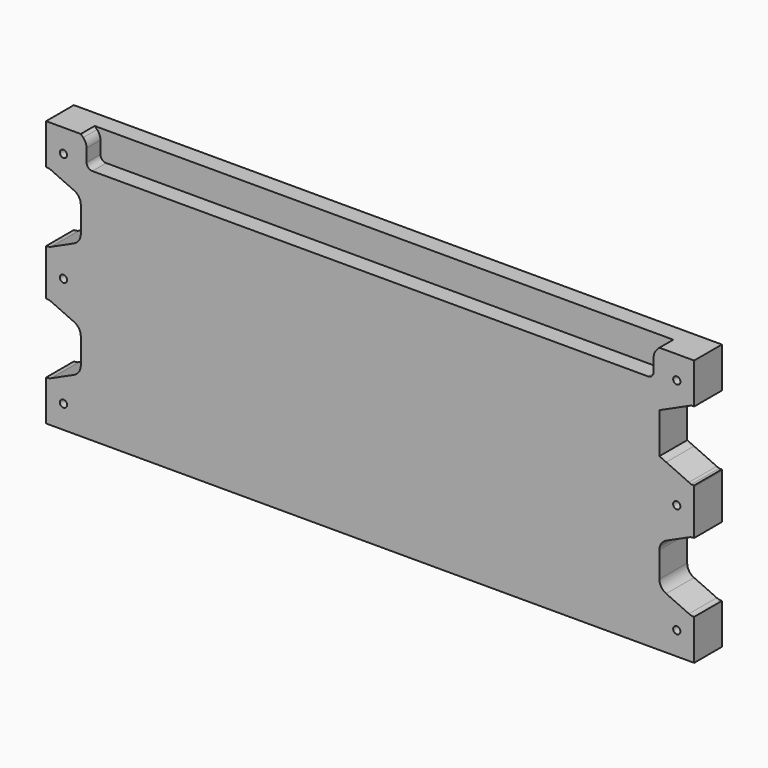
from build123d import *

# Parameters (mm, degrees)
F0_R     = 1.984375
F1_DEPTH = 9.525
F2_DEPTH = 9.525
F3_SIZE  = 3.175
F4_R     = 6.35


# Not quite as in the source:
# - ends of sketch curves that miss each other by under 0.0002 mm in the source are joined


with BuildPart() as f1:
    # F0 (on Front) → F1 (new body)
    with BuildSketch(Plane.XZ):
        with BuildLine():
            ThreePointArc((106.6892375248, 39.5968594302), (108.9343015551, 40.5267953999), (109.8642375248, 42.7718594302))
            Line((109.8642375248, 42.7718594302), (109.8642375248, 55.4718594302))
            Line((109.8642375248, 55.4718594302), (-201.2857624752, 55.4718594302))
            Line((-201.2857624752, 55.4718594302), (-201.2857624752, 42.7718594302))
            ThreePointArc((-201.2857624752, 42.7718594302), (-200.3558265055, 40.5267953999), (-198.1107624752, 39.5968594302))
            Line((-198.1107624752, 39.5968594302), (106.6892375248, 39.5968594302))
        make_face()
        with BuildLine():
            Line((109.8642375248, 55.4718594302), (109.8642375248, 42.7718594302))
            ThreePointArc((109.8642375248, 42.7718594302), (108.9343015551, 40.5267953999), (106.6892375248, 39.5968594302))
            Line((106.6892375248, 39.5968594302), (-198.1107624752, 39.5968594302))
            ThreePointArc((-198.1107624752, 39.5968594302), (-200.3558265055, 40.5267953999), (-201.2857624752, 42.7718594302))
            Line((-201.2857624752, 42.7718594302), (-201.2857624752, 55.4718594302))
            Line((-201.2857624752, 55.4718594302), (-223.5107624752, 55.4718594302))
            Line((-223.5107624752, 55.4718594302), (-223.5107624752, 33.2468594302))
            Line((-223.5107624752, 33.2468594302), (-223.2986885503, 33.2468594302))
            ThreePointArc((-223.2986885503, 33.2468594302), (-221.9543922864, 33.1029344825), (-220.6710339026, 32.6776838569))
            Line((-220.6710339026, 32.6776838569), (-208.1831078275, 27.0013383101))
            ThreePointArc((-208.1831078275, 27.0013383101), (-205.471843717, 24.6583106333), (-204.4607624752, 21.2205138834))
            Line((-204.4607624752, 21.2205138834), (-204.4607624752, 7.1731958926))
            ThreePointArc((-204.4607624752, 7.1731958926), (-205.4718446589, 3.7353976799), (-208.1831109951, 1.392370026))
            Line((-208.1831109951, 1.392370026), (-220.6710352489, -4.2839664363))
            ThreePointArc((-220.6710352489, -4.2839664363), (-221.9543921654, -4.7092159904), (-223.298686729, -4.8531405698))
            Line((-223.298686729, -4.8531405698), (-223.5107370752, -4.8531405698))
            Line((-223.5107370752, -4.8531405698), (-223.5107624752, -30.2531405698))
            Line((-223.5107624752, -30.2531405698), (-223.298686729, -30.2531405698))
            ThreePointArc((-223.298686729, -30.2531405698), (-221.9543921654, -30.3970651492), (-220.6710352489, -30.8223147033))
            Line((-220.6710352489, -30.8223147033), (-208.1831109951, -36.4986511657))
            ThreePointArc((-208.1831109951, -36.4986511657), (-205.4718446589, -38.8416788196), (-204.4607624752, -42.2794770322))
            Line((-204.4607624752, -42.2794770322), (-204.4607624752, -56.326795023))
            ThreePointArc((-204.4607624752, -56.326795023), (-205.471843717, -59.7645917729), (-208.1831078275, -62.1076194497))
            Line((-208.1831078275, -62.1076194497), (-220.6710339026, -67.7839649965))
            ThreePointArc((-220.6710339026, -67.7839649965), (-221.9543922864, -68.2092156221), (-223.2986885503, -68.3531405698))
            Line((-223.2986885503, -68.3531405698), (-223.5107370752, -68.3531405698))
            Line((-223.5107370752, -68.3531405698), (-223.5107624752, -90.5781405698))
            Line((-223.5107624752, -90.5781405698), (132.0892375248, -90.5781405698))
            Line((132.0892375248, -90.5781405698), (132.0892375248, -68.3531405698))
            Line((132.0892375248, -68.3531405698), (131.8771635999, -68.3531405698))
            ThreePointArc((131.8771635999, -68.3531405698), (130.532867336, -68.2092156221), (129.2495089522, -67.7839649965))
            Line((129.2495089522, -67.7839649965), (116.7615828771, -62.1076194497))
            ThreePointArc((116.7615828771, -62.1076194497), (114.0503187666, -59.7645917729), (113.0392375248, -56.326795023))
            Line((113.0392375248, -56.326795023), (113.0392375248, -42.2794770322))
            ThreePointArc((113.0392375248, -42.2794770322), (114.0503197085, -38.8416788196), (116.7615860447, -36.4986511657))
            Line((116.7615860447, -36.4986511657), (129.2495102985, -30.8223147033))
            ThreePointArc((129.2495102985, -30.8223147033), (130.5328672149, -30.3970651492), (131.8771617786, -30.2531405698))
            Line((131.8771617786, -30.2531405698), (132.0892121248, -30.2531405698))
            Line((132.0892121248, -30.2531405698), (132.0892375248, -5.5747531892))
            Line((132.0892375248, -5.5747531892), (130.5016917914, -4.8531405698))
            Line((130.5016917914, -4.8531405698), (129.2495102985, -4.2839664363))
            Line((129.2495102985, -4.2839664363), (116.7615860447, 1.392370026))
            Line((116.7615860447, 1.392370026), (113.0392375248, 3.0843487889))
            Line((113.0392375248, 3.0843487889), (113.0392375248, 7.1731958926))
            Line((113.0392375248, 7.1731958926), (113.0392375248, 21.2205138834))
            Line((113.0392375248, 21.2205138834), (113.0392375248, 25.3093700715))
            Line((113.0392375248, 25.3093700715), (116.7615794549, 27.001345839))
            Line((116.7615794549, 27.001345839), (129.2495086403, 32.677684543))
            Line((129.2495086403, 32.677684543), (130.5016917914, 33.2468594302))
            Line((130.5016917914, 33.2468594302), (132.0892375248, 33.9684720496))
            Line((132.0892375248, 33.9684720496), (132.0892375248, 55.4718594302))
            Line((132.0892375248, 55.4718594302), (109.8642375248, 55.4718594302))
        make_face()
        with Locations((-213.9857624752, -77.8781405698)):
            Circle(F0_R, mode=Mode.SUBTRACT)
        with Locations((122.5642375248, -77.8781405698)):
            Circle(F0_R, mode=Mode.SUBTRACT)
        with Locations((-213.9857624752, -17.5531402737)):
            Circle(F0_R, mode=Mode.SUBTRACT)
        with Locations((-213.9857624752, 42.7718594302)):
            Circle(F0_R, mode=Mode.SUBTRACT)
        with Locations((122.5642375248, -17.5531402737)):
            Circle(F0_R, mode=Mode.SUBTRACT)
        with Locations((122.5642375248, 42.7718594302)):
            Circle(F0_R, mode=Mode.SUBTRACT)
        Polygon((132.0892375248, 33.2468594302), (132.0892375248, 33.9684720496), (130.5016917914, 33.2468594302), (131.8771635999, 33.2468594302), align=None)
        Polygon((132.0892375248, -5.5747531892), (132.0892375248, -4.8531405698), (131.8771617786, -4.8531405698), (130.5016917914, -4.8531405698), align=None)
    extrude(amount=-F1_DEPTH)

    # F0 (on Front) → F2 (join)
    with BuildSketch(Plane.XZ):
        with BuildLine():
            Line((109.8642375248, 55.4718594302), (109.8642375248, 42.7718594302))
            ThreePointArc((109.8642375248, 42.7718594302), (108.9343015551, 40.5267953999), (106.6892375248, 39.5968594302))
            Line((106.6892375248, 39.5968594302), (-198.1107624752, 39.5968594302))
            ThreePointArc((-198.1107624752, 39.5968594302), (-200.3558265055, 40.5267953999), (-201.2857624752, 42.7718594302))
            Line((-201.2857624752, 42.7718594302), (-201.2857624752, 55.4718594302))
            Line((-201.2857624752, 55.4718594302), (-223.5107624752, 55.4718594302))
            Line((-223.5107624752, 55.4718594302), (-223.5107624752, 33.2468594302))
            Line((-223.5107624752, 33.2468594302), (-223.2986885503, 33.2468594302))
            ThreePointArc((-223.2986885503, 33.2468594302), (-221.9543922864, 33.1029344825), (-220.6710339026, 32.6776838569))
            Line((-220.6710339026, 32.6776838569), (-208.1831078275, 27.0013383101))
            ThreePointArc((-208.1831078275, 27.0013383101), (-205.471843717, 24.6583106333), (-204.4607624752, 21.2205138834))
            Line((-204.4607624752, 21.2205138834), (-204.4607624752, 7.1731958926))
            ThreePointArc((-204.4607624752, 7.1731958926), (-205.4718446589, 3.7353976799), (-208.1831109951, 1.392370026))
            Line((-208.1831109951, 1.392370026), (-220.6710352489, -4.2839664363))
            ThreePointArc((-220.6710352489, -4.2839664363), (-221.9543921654, -4.7092159904), (-223.298686729, -4.8531405698))
            Line((-223.298686729, -4.8531405698), (-223.5107370752, -4.8531405698))
            Line((-223.5107370752, -4.8531405698), (-223.5107624752, -30.2531405698))
            Line((-223.5107624752, -30.2531405698), (-223.298686729, -30.2531405698))
            ThreePointArc((-223.298686729, -30.2531405698), (-221.9543921654, -30.3970651492), (-220.6710352489, -30.8223147033))
            Line((-220.6710352489, -30.8223147033), (-208.1831109951, -36.4986511657))
            ThreePointArc((-208.1831109951, -36.4986511657), (-205.4718446589, -38.8416788196), (-204.4607624752, -42.2794770322))
            Line((-204.4607624752, -42.2794770322), (-204.4607624752, -56.326795023))
            ThreePointArc((-204.4607624752, -56.326795023), (-205.471843717, -59.7645917729), (-208.1831078275, -62.1076194497))
            Line((-208.1831078275, -62.1076194497), (-220.6710339026, -67.7839649965))
            ThreePointArc((-220.6710339026, -67.7839649965), (-221.9543922864, -68.2092156221), (-223.2986885503, -68.3531405698))
            Line((-223.2986885503, -68.3531405698), (-223.5107370752, -68.3531405698))
            Line((-223.5107370752, -68.3531405698), (-223.5107624752, -90.5781405698))
            Line((-223.5107624752, -90.5781405698), (132.0892375248, -90.5781405698))
            Line((132.0892375248, -90.5781405698), (132.0892375248, -68.3531405698))
            Line((132.0892375248, -68.3531405698), (131.8771635999, -68.3531405698))
            ThreePointArc((131.8771635999, -68.3531405698), (130.532867336, -68.2092156221), (129.2495089522, -67.7839649965))
            Line((129.2495089522, -67.7839649965), (116.7615828771, -62.1076194497))
            ThreePointArc((116.7615828771, -62.1076194497), (114.0503187666, -59.7645917729), (113.0392375248, -56.326795023))
            Line((113.0392375248, -56.326795023), (113.0392375248, -42.2794770322))
            ThreePointArc((113.0392375248, -42.2794770322), (114.0503197085, -38.8416788196), (116.7615860447, -36.4986511657))
            Line((116.7615860447, -36.4986511657), (129.2495102985, -30.8223147033))
            ThreePointArc((129.2495102985, -30.8223147033), (130.5328672149, -30.3970651492), (131.8771617786, -30.2531405698))
            Line((131.8771617786, -30.2531405698), (132.0892121248, -30.2531405698))
            Line((132.0892121248, -30.2531405698), (132.0892375248, -5.5747531892))
            Line((132.0892375248, -5.5747531892), (130.5016917914, -4.8531405698))
            Line((130.5016917914, -4.8531405698), (129.2495102985, -4.2839664363))
            Line((129.2495102985, -4.2839664363), (116.7615860447, 1.392370026))
            Line((116.7615860447, 1.392370026), (113.0392375248, 3.0843487889))
            Line((113.0392375248, 3.0843487889), (113.0392375248, 7.1731958926))
            Line((113.0392375248, 7.1731958926), (113.0392375248, 21.2205138834))
            Line((113.0392375248, 21.2205138834), (113.0392375248, 25.3093700715))
            Line((113.0392375248, 25.3093700715), (116.7615794549, 27.001345839))
            Line((116.7615794549, 27.001345839), (129.2495086403, 32.677684543))
            Line((129.2495086403, 32.677684543), (130.5016917914, 33.2468594302))
            Line((130.5016917914, 33.2468594302), (132.0892375248, 33.9684720496))
            Line((132.0892375248, 33.9684720496), (132.0892375248, 55.4718594302))
            Line((132.0892375248, 55.4718594302), (109.8642375248, 55.4718594302))
        make_face()
        with Locations((-213.9857624752, -77.8781405698)):
            Circle(F0_R, mode=Mode.SUBTRACT)
        with Locations((122.5642375248, -77.8781405698)):
            Circle(F0_R, mode=Mode.SUBTRACT)
        with Locations((-213.9857624752, -17.5531402737)):
            Circle(F0_R, mode=Mode.SUBTRACT)
        with Locations((-213.9857624752, 42.7718594302)):
            Circle(F0_R, mode=Mode.SUBTRACT)
        with Locations((122.5642375248, -17.5531402737)):
            Circle(F0_R, mode=Mode.SUBTRACT)
        with Locations((122.5642375248, 42.7718594302)):
            Circle(F0_R, mode=Mode.SUBTRACT)
        Polygon((132.0892375248, 33.2468594302), (132.0892375248, 33.9684720496), (130.5016917914, 33.2468594302), (131.8771635999, 33.2468594302), align=None)
        Polygon((132.0892375248, -5.5747531892), (132.0892375248, -4.8531405698), (131.8771617786, -4.8531405698), (130.5016917914, -4.8531405698), align=None)
    extrude(amount=F2_DEPTH)

    # F3
    f3_edges = [f1.edges().sort_by_distance(p)[0] for p in [
        (-201.285762, -4.7625, 55.471859),
        (109.864238, -4.7625, 55.471859),
    ]]
    chamfer(f3_edges, length=F3_SIZE)

    # F4
    f4_edges = [f1.edges().sort_by_distance(p)[0] for p in [
        (109.864238, -4.7625, 52.296859),
        (-201.285762, -4.7625, 52.296859),
    ]]
    fillet(f4_edges, radius=F4_R)


solid = f1.part
